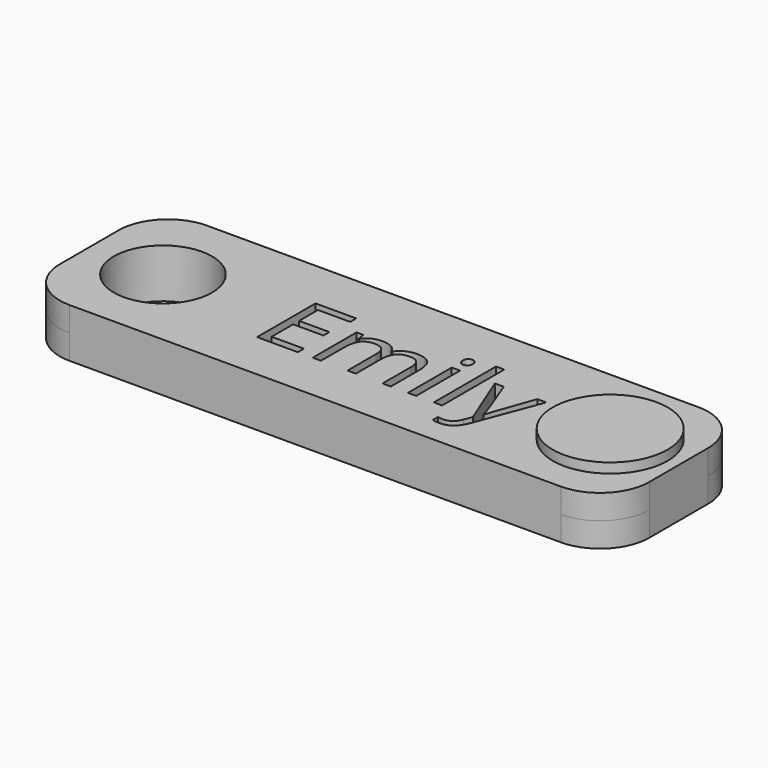
from build123d import *

# Parameters (mm, degrees)
F0_W         = 120
F0_H         = 35
F0_R         = 10
F1_DEPTH     = 5
F2_R         = 10
F3_TEXT_SIZE = 20.8333333333
F4_DEPTH     = 2
F5_W         = 1.689453125
F5_H         = 11.1490885417
F5_R         = 10
F5_H_2       = 15.830078125
F6_DEPTH     = 5
F7_R         = 11.6886860398
F8_DEPTH     = 2


# Not quite as in the source:
# - Text() gives the source's letters only with a copy of the font that has no kerning and outlines rounded to 1/6400 em; it was checked with that copy


with BuildPart() as f1:
    # F0 (on Top) → F1 (new body)
    with BuildSketch(Plane.XY):
        Rectangle(F0_W, F0_H)
        with Locations((-45, 0)):
            Circle(F0_R, mode=Mode.SUBTRACT)
    extrude(amount=F1_DEPTH)

    # F2
    f2_edges = [f1.edges().sort_by_distance(p)[0] for p in [
        (-60, -17.5, 2.5),
        (60, -17.5, 2.5),
        (-60, 17.5, 2.5),
        (60, 17.5, 2.5),
    ]]
    fillet(f2_edges, radius=F2_R)

    # F3 (on face) → F4 (join)
    with BuildSketch(Plane.XY.offset(5)):
        with Locations((-21.8852456968, -7.5)):
            Text('Emily', F3_TEXT_SIZE, font='Open Sans', text_align=(TextAlign.LEFT, TextAlign.BOTTOM))
    extrude(amount=F4_DEPTH)

    # F5 (on face) → F6 (join)
    with BuildSketch(Plane.XY.offset(5)):
        with BuildLine():
            ThreePointArc((-60, -7.5), (-57.0710678119, -14.5710678119), (-50, -17.5))
            Line((-50, -17.5), (50, -17.5))
            ThreePointArc((50, -17.5), (57.0710678119, -14.5710678119), (60, -7.5))
            Line((60, -7.5), (60, 7.5))
            ThreePointArc((60, 7.5), (57.0710678119, 14.5710678119), (50, 17.5))
            Line((50, 17.5), (-50, 17.5))
            ThreePointArc((-50, 17.5), (-57.0710678119, 14.5710678119), (-60, 7.5))
            Line((-60, 7.5), (-60, -7.5))
        make_face()
        Polygon((-11.5499592385, -5.9537760417), (-11.5499592385, -7.5), (-19.8409748635, -7.5), (-19.8409748635, 7.373046875), (-11.5499592385, 7.373046875), (-11.5499592385, 5.8365885417), (-18.1124592385, 5.8365885417), (-18.1124592385, 1.044921875), (-11.9470946552, 1.044921875), (-11.9470946552, -0.4817708333), (-18.1124592385, -0.4817708333), (-18.1124592385, -5.9537760417), align=None, mode=Mode.SUBTRACT)
        with BuildLine():
            Line((7.3888428448, -7.5), (5.7026449282, -7.5))
            Line((5.7026449282, -7.5), (5.7026449282, -0.2473958333))
            add(Edge.make_bspline(
                [(0.2794678448, -1.2727864583), (0.2794678448, 0.6087239583), (1.7866293032, 2.4186197917), (4.5633220115, 2.4186197917), (5.7026449282, 1.0872395833), (5.7026449282, -0.2473958333)],
                knots=[0, 0, 0, 1, 2, 2.7623966942, 3.5247933884, 3.5247933884, 3.5247933884], degree=2))
            Line((0.2794678448, -1.2727864583), (0.2794678448, -7.5))
            Line((0.2794678448, -7.5), (-1.4099852802, -7.5))
            Line((-1.4099852802, -7.5), (-1.4099852802, -0.2473958333))
            add(Edge.make_bspline(
                [(-6.8201415302, -1.650390625), (-6.8201415302, 0.517578125), (-5.3455321552, 2.4186197917), (-2.5493081968, 2.4186197917), (-1.4099852802, 1.0872395833), (-1.4099852802, -0.2473958333)],
                knots=[0, 0, 0, 1, 2, 2.7638603696, 3.5277207392, 3.5277207392, 3.5277207392], degree=2))
            Line((-6.8201415302, -1.650390625), (-6.8201415302, -7.5))
            Line((-6.8201415302, -7.5), (-8.5095946552, -7.5))
            Line((-8.5095946552, -7.5), (-8.5095946552, 3.6490885417))
            Line((-8.5095946552, 3.6490885417), (-7.1358967385, 3.6490885417))
            Line((-7.1358967385, 3.6490885417), (-6.8624592385, 2.1223958333))
            Line((-6.8624592385, 2.1223958333), (-6.7810790302, 2.1223958333))
            add(Edge.make_bspline(
                [(-0.0655842385, 1.9596354167), (-0.8696206968, 3.8541666667), (-4.5610269468, 3.8541666667), (-6.3025634052, 2.9361979167), (-6.7810790302, 2.1223958333)],
                knots=[0, 0, 0, 1, 1.4122042341, 1.8244084682, 1.8244084682, 1.8244084682], degree=2))
            Line((-0.0655842385, 1.9596354167), (0.0157959698, 1.9596354167))
            add(Edge.make_bspline(
                [(7.3888428448, -0.2278645833), (7.3888428448, 1.9108072917), (5.5073324282, 3.8541666667), (2.4051188865, 3.8541666667), (0.5138428448, 2.8352864583), (0.0157959698, 1.9596354167)],
                knots=[0, 0, 0, 1, 2, 2.6402753873, 3.2805507745, 3.2805507745, 3.2805507745], degree=2))
            Line((7.3888428448, -0.2278645833), (7.3888428448, -7.5))
        make_face(mode=Mode.SUBTRACT)
        with BuildLine():
            Line((28.2872803448, 3.6490885417), (30.0971761782, 3.6490885417))
            Line((30.0971761782, 3.6490885417), (25.3055095115, -9.0462239583))
            add(Edge.make_bspline(
                [(19.7814209698, -12.3307291667), (20.5333740948, -12.5065104167), (22.6915772198, -12.5065104167), (24.5926188865, -10.927734375), (25.3055095115, -9.0462239583)],
                knots=[0, 0, 0, 1, 2.7857142857, 4.5714285714, 4.5714285714, 4.5714285714], degree=2))
            Line((19.7814209698, -12.3307291667), (19.7814209698, -10.9798177083))
            add(Edge.make_bspline(
                [(23.5151449282, -9.1471354167), (22.7729574282, -11.1002604167), (20.3413168032, -11.1002604167), (19.7814209698, -10.9798177083)],
                knots=[0, 0, 0, 1, 1.3962616822, 1.3962616822, 1.3962616822], degree=2))
            Line((23.5151449282, -9.1471354167), (24.1368897198, -7.5618489583))
            Line((24.1368897198, -7.5618489583), (19.6381918032, 3.6490885417))
            Line((19.6381918032, 3.6490885417), (21.4513428448, 3.6490885417))
            Line((21.4513428448, 3.6490885417), (23.8927490948, -2.7083333333))
            add(Edge.make_bspline(
                [(23.8927490948, -2.7083333333), (24.6935303448, -4.8860677083), (24.8888428448, -5.8528645833)],
                knots=[0, 0, 0, 1, 1, 1], degree=2))
            Line((24.8888428448, -5.8528645833), (24.9702230532, -5.8528645833))
            add(Edge.make_bspline(
                [(28.2872803448, 3.6490885417), (25.9467855532, -2.8190104167), (25.1004313865, -5.33203125), (24.9702230532, -5.8528645833)],
                knots=[0, 0, 0, 1, 2, 2, 2], degree=2))
        make_face(mode=Mode.SUBTRACT)
        with Locations((11.7133871157, -1.9254557292)):
            Rectangle(F5_W, F5_H, mode=Mode.SUBTRACT)
        with Locations((-45, 0)):
            Circle(F5_R, mode=Mode.SUBTRACT)
        with Locations((16.9835694073, 0.4150390625)):
            Rectangle(F5_W, F5_H_2, mode=Mode.SUBTRACT)
        with BuildLine():
            add(Edge.make_bspline(
                [(10.7254313865, 6.669921875), (10.7254313865, 6.1002604167), (11.2950928448, 5.5403645833), (12.1316813865, 5.5403645833), (12.7208740948, 6.1002604167), (12.7208740948, 7.2395833333), (12.1316813865, 7.7897135417), (11.2950928448, 7.7897135417), (10.7254313865, 7.2493489583), (10.7254313865, 6.669921875)],
                knots=[0, 0, 0, 1, 2, 2.946969697, 3.8939393939, 4.8409090909, 5.7878787879, 6.7878787879, 7.7878787879, 7.7878787879, 7.7878787879], degree=2))
        make_face(mode=Mode.SUBTRACT)
    extrude(amount=F6_DEPTH)

    # F7 (on face) → F8 (join)
    with BuildSketch(Plane.XY.offset(10)):
        with Locations((46.0474863648, 0)):
            Circle(F7_R)
    extrude(amount=F8_DEPTH)


solid = f1.part
